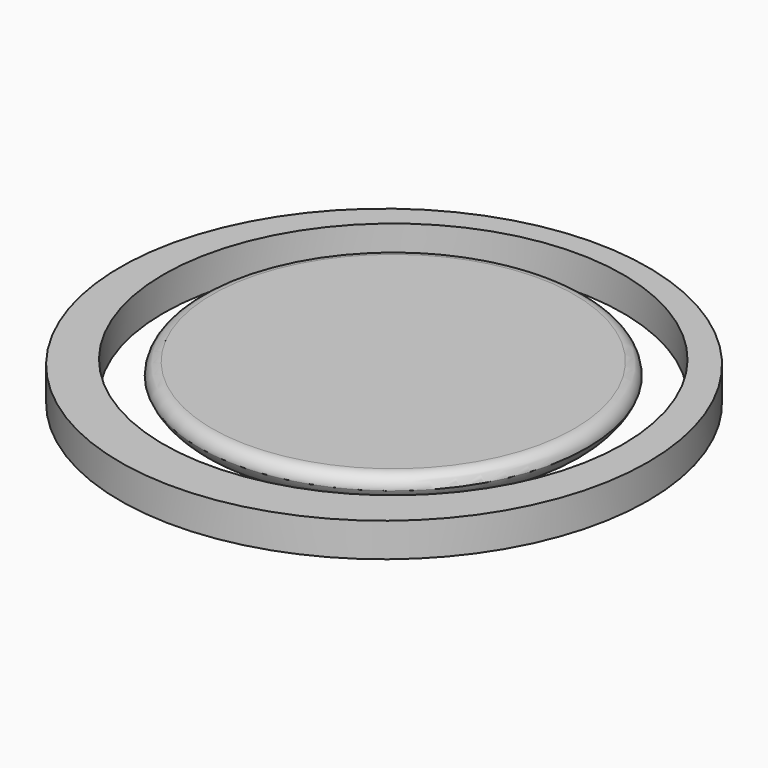
from build123d import *

# Parameters (mm, degrees)
F0_R     = 30.3340575797
F1_DEPTH = 5
F2_R     = 2
F4_R     = 41.2533832891
F4_R_2   = 35.9200098551
F5_DEPTH = 5.3


# Not quite as in the source:
# - a fillet or chamfer that OpenCascade refuses, or shapes differently, is made with other operations: its cross-section is extruded or revolved along the edge and cut away or added


with BuildPart() as f1:
    # F0 (on Top) → F1 (new body)
    with BuildSketch(Plane.XY):
        Circle(F0_R)
    extrude(amount=F1_DEPTH)

    # F2
    f2_edges = [f1.edges().sort_by_distance(p)[0] for p in [
        (-30.334058, 0, 5),
    ]]
    fillet(f2_edges, radius=F2_R)

    # F3: fillet of radius 5 on 3 edges, made by hand

    # F3_s1 → F3_t2 (revolve, cut)
    with BuildSketch(Plane.XZ):
        with BuildLine():
            ThreePointArc((30.3340575797, 3), (28.4900946723, 0.8166998673), (25.7514818848, 0))
            Line((25.7514818848, 0), (25.7514818848, -0.1))
            Line((25.7514818848, -0.1), (30.3340575797, -0.1))
            Line((30.3340575797, -0.1), (30.4340575797, 0))
            ThreePointArc((30.4340575797, 0), (30.4340575797, 1.5), (30.4257090936, 2.96))
            Line((30.4257090936, 2.96), (30.3340575797, 3))
        make_face()
    revolve(axis=Axis((0, 0, 0), (0, 0, 1)), mode=Mode.SUBTRACT)


with BuildPart() as f5:
    # F4 (on Top) → F5 (new body)
    with BuildSketch(Plane.XY):
        with Locations((0, -1.7924887361)):
            Circle(F4_R)
        Circle(F4_R_2, mode=Mode.SUBTRACT)
    extrude(amount=F5_DEPTH)


solid = Compound([f1.part, f5.part])
